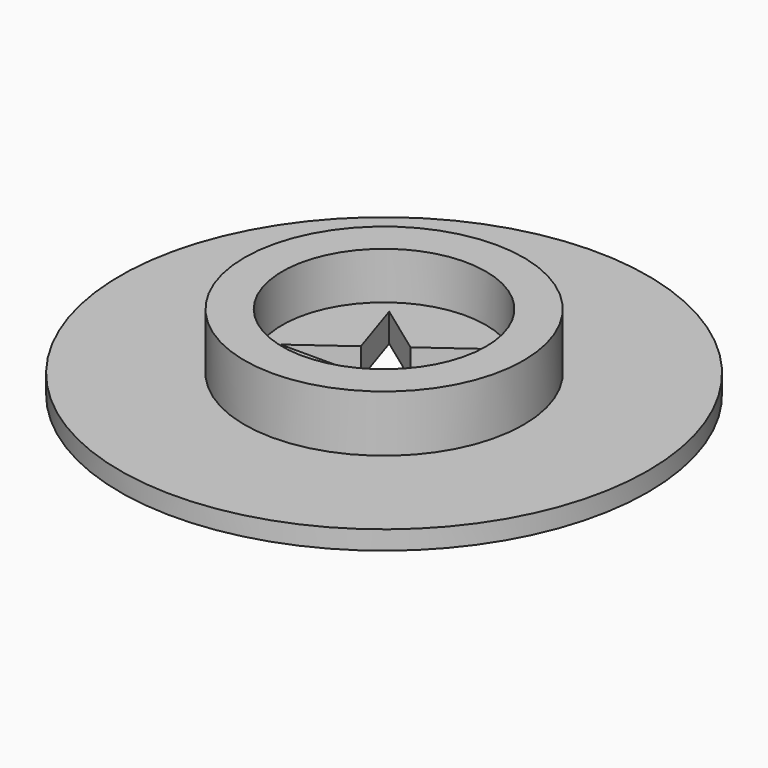
from build123d import *

# Parameters (mm, degrees)
F3_DEPTH = 25


with BuildPart() as f1:
    # F0 (on Front) → F1 (revolve)
    with BuildSketch(Plane.XZ):
        Polygon((0, 1.5), (0, 0), (14, 0), (14, 1), (7.4, 1), (7.4, 4), (5.4, 4), (5.4, 1.5), align=None)
    revolve(axis=Axis((0, 0, 0.75), (0, 0, -1)))

    # F2 (on face) → F3 (cut)
    with BuildSketch(Plane.XY.offset(1.5)):
        Polygon((-1.0285587608, -1.4156896825), (-1.6642430343, 0.5407453412), (-4.3570448294, -1.4156896825), align=None)
        Polygon((0, 1.7498886826), (-2.6928017951, 3.7063237062), (-1.6642430343, 0.5407453412), align=None)
        Polygon((1.6642430343, 0.5407453412), (0, 1.7498886826), (-1.6642430343, 0.5407453412), (-1.0285587608, -1.4156896825), (1.0285587608, -1.4156896825), align=None)
        Polygon((2.6928017951, 3.7063237062), (0, 1.7498886826), (1.6642430343, 0.5407453412), align=None)
        Polygon((4.3570448294, -1.4156896825), (1.6642430343, 0.5407453412), (1.0285587608, -1.4156896825), align=None)
        Polygon((1.0285587608, -1.4156896825), (-1.0285587608, -1.4156896825), (0, -4.5812680475), align=None)
    extrude(amount=-F3_DEPTH, mode=Mode.SUBTRACT)


solid = f1.part
